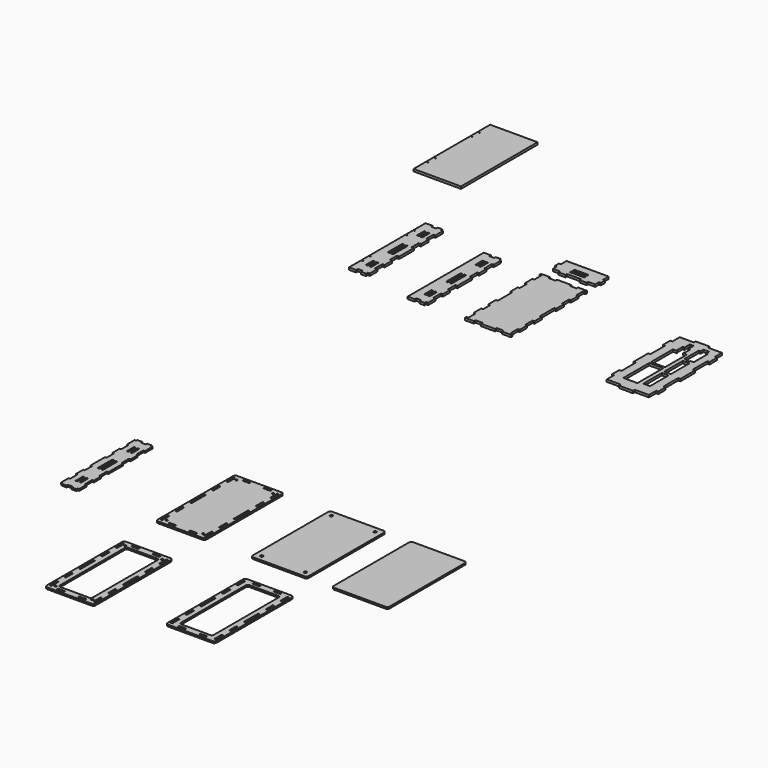
from build123d import *

# Parameters (mm, degrees)
F0_R     = 1.5
F1_DEPTH = 6.33
F0_W     = 40
F0_H     = 5.2
F0_H_2   = 92
F0_W_2   = 19
F0_H_3   = 66
F0_W_3   = 5.2
F0_H_4   = 26
F0_H_5   = 52
F0_R_2   = 2.8
F0_W_4   = 4.5
F0_H_6   = 25.7
F0_H_7   = 25.4
F2_DEPTH = 5
F0_R_3   = 3.8


# Not quite as in the source:
# - ends of sketch curves that miss each other by under 0.0002 mm in the source are joined


with BuildPart() as f1:
    # F0 (on Top) → F1 (new body)
    with BuildSketch(Plane.XY):
        Polygon((-447.6903581619, 704.729092989), (-582.6903581619, 704.729092989), (-582.6903581619, 660.318092989), (-582.6903581619, 432.069092989), (-447.6903581619, 432.069092989), (-447.6903581619, 568.399092989), align=None)
        with Locations((-577.6903581619, 476.480092989)):
            Circle(F0_R, mode=Mode.SUBTRACT)
        with Locations((-577.4039030075, 503.1310149765)):
            Circle(F0_R, mode=Mode.SUBTRACT)
        with BuildLine():
            ThreePointArc((-577.6903581619, 635.218092989), (-576.6296979901, 634.7787531607), (-576.1903581619, 633.718092989))
            ThreePointArc((-576.1903581619, 633.718092989), (-578.7510183337, 632.6574328172), (-577.6903581619, 635.218092989))
        make_face(mode=Mode.SUBTRACT)
        with BuildLine():
            ThreePointArc((-577.6903581619, 658.818092989), (-578.7510183337, 659.2574328172), (-579.1903581619, 660.318092989))
            ThreePointArc((-579.1903581619, 660.318092989), (-577.6903581619, 661.818092989), (-576.1903581619, 660.318092989))
            ThreePointArc((-576.1903581619, 660.318092989), (-576.6296979901, 659.2574328172), (-577.6903581619, 658.818092989))
        make_face(mode=Mode.SUBTRACT)
    extrude(amount=F1_DEPTH)


with BuildPart() as f1b:
    # F0 (on Top) → F1, piece 2 (new body)
    with BuildSketch(Plane.XY):
        Polygon((-0.3, 209.1742812097), (-19.7, 209.1742812097), (-19.7, 214.6742812097), (-45.5, 214.6742812097), (-45.5, 209.1742812097), (-40, 209.1742812097), (-40, 183.4742812097), (-45.5, 183.4742812097), (-45.5, 156.8742812097), (-40, 156.8742812097), (-40, 131.4742812097), (-45.5, 131.4742812097), (-45.5, 104.8742812097), (-40, 104.8742812097), (-40, 79.1742812097), (-40, 53.4742812097), (-45.5, 53.4742812097), (-45.5, 26.8742812097), (-40, 26.8742812097), (-40, 1.4742812097), (-45.5, 1.4742812097), (-45.5, -25.1257187903), (-40, -25.1257187903), (-40, -50.8257187903), (-45.5, -50.8257187903), (-45.5, -56.3257187903), (-19.7, -56.3257187903), (-19.7, -50.8257187903), (-0.3, -50.8257187903), (-0.3, -56.3257187903), (20, -56.3257187903), (40.3, -56.3257187903), (40.3, -50.8257187903), (59.7, -50.8257187903), (59.7, -56.3257187903), (85.5, -56.3257187903), (85.5, -50.8257187903), (80, -50.8257187903), (80, -25.1257187903), (85.5, -25.1257187903), (85.5, 1.4742812097), (80, 1.4742812097), (80, 26.8742812097), (85.5, 26.8742812097), (85.5, 53.4742812097), (80, 53.4742812097), (80, 79.1742812097), (80, 104.8742812097), (85.5, 104.8742812097), (85.5, 131.4742812097), (80, 131.4742812097), (80, 156.8742812097), (85.5, 156.8742812097), (85.5, 183.4742812097), (80, 183.4742812097), (80, 209.1742812097), (85.5, 209.1742812097), (85.5, 214.6742812097), (59.7, 214.6742812097), (59.7, 209.1742812097), (40.3, 209.1742812097), (40.3, 214.6742812097), (20, 214.6742812097), (-0.3, 214.6742812097), align=None)
    extrude(amount=F1_DEPTH)


with BuildPart() as f1c:
    # F0 (on Top) → F1, piece 3 (new body)
    with BuildSketch(Plane.XY):
        Polygon((-40, 263.7736713409), (-40, 250.0736713409), (-20.3, 250.0736713409), (-20, 250.0736713409), (-20, 244.5736713409), (0, 244.5736713409), (0, 250.0736713409), (0.3, 250.0736713409), (20, 250.0736713409), (39.7, 250.0736713409), (40, 250.0736713409), (40, 244.5736713409), (44.012218684, 244.5736713409), (60, 244.5736713409), (60, 250.0736713409), (60.3, 250.0736713409), (80, 250.0736713409), (80, 263.7736713409), (85.5, 263.7736713409), (85.5, 278.3736713409), (80, 278.3736713409), (80, 292.0736713409), (80, 298.4036713409), (60, 298.4036713409), (40, 298.4036713409), (0, 298.4036713409), (-20, 298.4036713409), (-40, 298.4036713409), (-40, 292.0736713409), (-40, 278.3736713409), (-45.5, 278.3736713409), (-45.5, 263.7736713409), align=None)
        with Locations((20, 263.6386713409)):
            Rectangle(F0_W, F0_H, mode=Mode.SUBTRACT)
        with Locations((20, 273.8386713409)):
            Rectangle(F0_W, F0_H, mode=Mode.SUBTRACT)
    extrude(amount=F1_DEPTH)


with BuildPart() as f1d:
    # F0 (on Top) → F1, piece 4 (new body)
    with BuildSketch(Plane.XY):
        Polygon((385.8841769994, -91.011034461), (405.8841769994, -91.011034461), (425.8841769994, -91.011034461), (425.8841769994, -97.341034461), (465.8841769994, -97.341034461), (465.8841769994, -91.011034461), (485.8841769994, -91.011034461), (505.8841769994, -91.011034461), (505.8841769994, -65.011034461), (512.2141769994, -65.011034461), (512.2141769994, -39.011034461), (505.8841769994, -39.011034461), (505.8841769994, -13.011034461), (505.8841769994, 12.988965539), (512.2141769994, 12.988965539), (512.2141769994, 64.988965539), (505.8841769994, 64.988965539), (505.8841769994, 90.988965539), (505.8841769994, 116.988965539), (512.2141769994, 116.988965539), (512.2141769994, 142.988965539), (505.8841769994, 142.988965539), (505.8841769994, 168.988965539), (485.8841769994, 168.988965539), (465.8841769994, 168.988965539), (465.8841769994, 175.318965539), (445.8841769994, 175.318965539), (425.8841769994, 175.318965539), (425.8841769994, 168.988965539), (405.8841769994, 168.988965539), (385.8841769994, 168.988965539), (385.8841769994, 142.988965539), (379.5541769994, 142.988965539), (379.5541769994, 116.988965539), (385.8841769994, 116.988965539), (385.8841769994, 90.988965539), (385.8841769994, 64.988965539), (379.5541769994, 64.988965539), (379.5541769994, 12.988965539), (385.8841769994, 12.988965539), (385.8841769994, -13.011034461), (385.8841769994, -39.011034461), (379.5541769994, -39.011034461), (379.5541769994, -65.011034461), (385.8841769994, -65.011034461), align=None)
        with Locations((430.4254828245, -16.4253961511)):
            Rectangle(F0_W, F0_H_2, mode=Mode.SUBTRACT)
        with Locations((471.857395351, -23.1853164307)):
            Rectangle(F0_W_2, F0_H_3, mode=Mode.SUBTRACT)
        Polygon((424.9906819054, 136.7675569632), (424.9906819054, 155.7675569632), (435.9906819054, 155.7675569632), (435.9906819054, 154.7675569632), (435.9906819054, 136.7675569632), (440.9906819054, 136.7675569632), (440.9906819054, 118.7675569632), (439.4906819054, 118.7675569632), (439.4906819054, 113.7675569632), (450.4906819054, 113.7675569632), (450.4906819054, 35.7675569632), (410.4906819054, 35.7675569632), (410.4906819054, 113.7675569632), (421.4906819054, 113.7675569632), (421.4906819054, 118.7675569632), (419.9906819054, 118.7675569632), (419.9906819054, 136.7675569632), align=None, mode=Mode.SUBTRACT)
        with Locations((471.857395351, 51.1568081991)):
            Rectangle(F0_W_2, F0_H_3, mode=Mode.SUBTRACT)
        Polygon((459.2148857416, 94.0252485254), (459.2148857416, 145.0252485254), (464.2148857416, 145.0252485254), (464.2148857416, 155.0252485254), (472.2148857416, 155.0252485254), (480.2148857416, 155.0252485254), (480.2148857416, 145.0252485254), (485.2148857416, 145.0252485254), (485.2148857416, 94.0252485254), (475.7148857416, 94.0252485254), (475.7148857416, 89.0252485254), (472.2148857416, 89.0252485254), (468.7148857416, 89.0252485254), (468.7148857416, 94.0252485254), align=None, mode=Mode.SUBTRACT)
    extrude(amount=F1_DEPTH)


with BuildPart() as f1e:
    # F0 (on Top) → F1, piece 5 (new body)
    with BuildSketch(Plane.XY):
        Polygon((-181.5613321495, 209.1742812097), (-188.5613321495, 209.1742812097), (-188.5613321495, 214.6742812097), (-208.8913321495, 214.6742812097), (-208.8913321495, 209.1742812097), (-208.8913321495, 183.1742812097), (-208.8913321495, 157.1742812097), (-208.8913321495, 79.1742812097), (-208.8913321495, 1.1742812097), (-208.8913321495, -24.8257187903), (-208.8913321495, -50.8257187903), (-208.8913321495, -56.3257187903), (-188.5613321495, -56.3257187903), (-188.5613321495, -50.8257187903), (-181.5613321495, -50.8257187903), (-174.8613321495, -50.8257187903), (-174.5613321495, -50.8257187903), (-174.5613321495, -56.3257187903), (-160.5613321495, -56.3257187903), (-160.5613321495, -50.8257187903), (-155.0613321495, -50.8257187903), (-155.0613321495, -24.8257187903), (-160.5613321495, -24.8257187903), (-160.5613321495, -24.5257187903), (-160.5613321495, 0.8742812097), (-160.5613321495, 1.1742812097), (-155.0613321495, 1.1742812097), (-155.0613321495, 27.1742812097), (-160.5613321495, 27.1742812097), (-160.5613321495, 27.4742812097), (-160.5613321495, 52.8742812097), (-160.5613321495, 53.1742812097), (-155.0613321495, 53.1742812097), (-155.0613321495, 79.1742812097), (-155.0613321495, 105.1742812097), (-160.5613321495, 105.1742812097), (-160.5613321495, 105.4742812097), (-160.5613321495, 130.8742812097), (-160.5613321495, 131.1742812097), (-155.0613321495, 131.1742812097), (-155.0613321495, 157.1742812097), (-160.5613321495, 157.1742812097), (-160.5613321495, 157.4742812097), (-160.5613321495, 182.8742812097), (-160.5613321495, 183.1742812097), (-155.0613321495, 183.1742812097), (-155.0613321495, 209.4742812097), (-160.2613321495, 209.4742812097), (-160.5613321495, 209.4742812097), (-160.5613321495, 214.6742812097), (-174.5613321495, 214.6742812097), (-174.5613321495, 209.1742812097), (-174.8613321495, 209.1742812097), align=None)
        Polygon((-184.7263321495, -24.8257187903), (-186.9263321495, -24.8257187903), (-186.9263321495, 1.1742812097), (-181.7263321495, 1.1742812097), (-181.7263321495, -24.8257187903), align=None, mode=Mode.SUBTRACT)
        with Locations((-174.1263321495, -11.8257187903)):
            Rectangle(F0_W_3, F0_H_4, mode=Mode.SUBTRACT)
        Polygon((-186.9263321495, 79.1742812097), (-186.9263321495, 105.1742812097), (-181.8263321495, 105.1742812097), (-181.8263321495, 79.1742812097), (-181.8263321495, 53.1742812097), (-186.9263321495, 53.1742812097), align=None, mode=Mode.SUBTRACT)
        Polygon((-176.7263321495, 105.1742812097), (-171.6263321495, 105.1742812097), (-171.6263321495, 79.1742812097), (-171.6263321495, 53.1742812097), (-176.7263321495, 53.1742812097), (-176.7263321495, 79.1742812097), align=None, mode=Mode.SUBTRACT)
        Polygon((-186.9263321495, 157.1742812097), (-186.9263321495, 183.1742812097), (-184.7263321495, 183.1742812097), (-181.7263321495, 183.1742812097), (-181.7263321495, 157.1742812097), align=None, mode=Mode.SUBTRACT)
        with Locations((-174.1263321495, 170.1742812097)):
            Rectangle(F0_W_3, F0_H_4, mode=Mode.SUBTRACT)
    extrude(amount=F1_DEPTH)


with BuildPart() as f1f:
    # F0 (on Top) → F1, piece 6 (new body)
    with BuildSketch(Plane.XY):
        Polygon((-371.3439686881, 239.1072111412), (-378.3439686881, 239.1072111412), (-378.3439686881, 244.8072111412), (-398.6739686881, 244.8072111412), (-398.6739686881, 239.1072111412), (-398.6739686881, 212.5072111412), (-398.6739686881, 200.4259941339), (-398.6739686881, 186.5072111412), (-398.6739686881, 173.8259941339), (-398.6739686881, -21.4927888588), (-398.6739686881, -27.8227888588), (-392.3439686881, -27.8227888588), (-378.3439686881, -27.8227888588), (-378.3439686881, -21.4927888588), (-364.6439686881, -21.4927888588), (-364.6439686881, -27.8227888588), (-364.3439686881, -27.8227888588), (-357.3439686881, -27.8227888588), (-350.3439686881, -27.8227888588), (-350.0439686881, -27.8227888588), (-350.0439686881, -21.4927888588), (-344.0139686881, -21.4927888588), (-344.0139686881, 4.5072111412), (-350.3439686881, 4.5072111412), (-350.3439686881, 4.8072111412), (-350.3439686881, 30.2072111412), (-350.3439686881, 30.5072111412), (-344.0139686881, 30.5072111412), (-344.0139686881, 56.5072111412), (-350.3439686881, 56.5072111412), (-350.3439686881, 56.8072111412), (-350.3439686881, 82.2072111412), (-350.3439686881, 82.5072111412), (-344.0139686881, 82.5072111412), (-344.0139686881, 108.5072111412), (-344.0139686881, 134.5072111412), (-350.3439686881, 134.5072111412), (-350.3439686881, 134.8072111412), (-350.3439686881, 159.6072111412), (-350.3439686881, 159.9072111412), (-344.0139686881, 159.9072111412), (-344.0139686881, 186.5072111412), (-350.3439686881, 186.5072111412), (-350.3439686881, 186.8072111412), (-350.3439686881, 212.5072111412), (-344.8439686881, 212.5072111412), (-344.8439686881, 239.1072111412), (-350.0439686881, 239.1072111412), (-350.3439686881, 239.1072111412), (-350.3439686881, 244.8072111412), (-364.3439686881, 244.8072111412), (-364.3439686881, 239.1072111412), (-364.6439686881, 239.1072111412), align=None)
        with Locations((-394.6739686881, 16.5884281485)):
            Circle(F0_R, mode=Mode.SUBTRACT)
        with Locations((-374.1089686881, 17.5072111412)):
            Rectangle(F0_W_3, F0_H_4, mode=Mode.SUBTRACT)
        with Locations((-394.6739686881, 43.1884281485)):
            Circle(F0_R, mode=Mode.SUBTRACT)
        with Locations((-363.9089686881, 17.5072111412)):
            Rectangle(F0_W_3, F0_H_4, mode=Mode.SUBTRACT)
        with Locations((-374.1089686881, 108.5072111412)):
            Rectangle(F0_W_3, F0_H_5, mode=Mode.SUBTRACT)
        with Locations((-363.9089686881, 108.5072111412)):
            Rectangle(F0_W_3, F0_H_5, mode=Mode.SUBTRACT)
        with BuildLine():
            ThreePointArc((-393.1739686881, 173.8259941339), (-394.6739686881, 172.3259941339), (-396.1739686881, 173.8259941339))
            ThreePointArc((-396.1739686881, 173.8259941339), (-395.7346288598, 174.8866543057), (-394.6739686881, 175.3259941339))
            ThreePointArc((-394.6739686881, 175.3259941339), (-393.6133085163, 174.8866543057), (-393.1739686881, 173.8259941339))
        make_face(mode=Mode.SUBTRACT)
        with BuildLine():
            ThreePointArc((-394.6739686881, 198.9259941339), (-395.7346288598, 199.3653339622), (-396.1739686881, 200.4259941339))
            ThreePointArc((-396.1739686881, 200.4259941339), (-394.6739686881, 201.9259941339), (-393.1739686881, 200.4259941339))
            ThreePointArc((-393.1739686881, 200.4259941339), (-393.6133085163, 199.3653339622), (-394.6739686881, 198.9259941339))
        make_face(mode=Mode.SUBTRACT)
        Polygon((-376.7089686881, 186.5072111412), (-376.7089686881, 212.5072111412), (-374.5089686881, 212.5072111412), (-371.5089686881, 212.5072111412), (-371.5089686881, 186.5072111412), align=None, mode=Mode.SUBTRACT)
        with Locations((-363.9089686881, 199.5072111412)):
            Rectangle(F0_W_3, F0_H_4, mode=Mode.SUBTRACT)
    extrude(amount=F1_DEPTH)


with BuildPart() as f2:
    # F0 (on Top) → F2 (new body)
    with BuildSketch(Plane.XY):
        with BuildLine():
            Line((26.3501927257, -971.6120737515), (26.3501927257, -1105.7620737515))
            Line((26.3501927257, -1105.7620737515), (26.3501927257, -1239.9120737515))
            ThreePointArc((26.3501927257, -1239.9120737515), (28.2100646651, -1244.402201812), (32.7001927257, -1246.2620737515))
            Line((32.7001927257, -1246.2620737515), (95.8501927257, -1246.2620737515))
            Line((95.8501927257, -1246.2620737515), (159.0001927257, -1246.2620737515))
            ThreePointArc((159.0001927257, -1246.2620737515), (163.4903207862, -1244.402201812), (165.3501927257, -1239.9120737515))
            Line((165.3501927257, -1239.9120737515), (165.3501927257, -1105.7620737515))
            Line((165.3501927257, -1105.7620737515), (165.3501927257, -971.6120737515))
            ThreePointArc((165.3501927257, -971.6120737515), (163.4903207862, -967.121945691), (159.0001927257, -965.2620737515))
            Line((159.0001927257, -965.2620737515), (95.8501927257, -965.2620737515))
            Line((95.8501927257, -965.2620737515), (32.7001927257, -965.2620737515))
            ThreePointArc((32.7001927257, -965.2620737515), (28.2100646651, -967.121945691), (26.3501927257, -971.6120737515))
        make_face()
        with Locations((43.6520688236, -1229.9456782266)):
            Circle(F0_R_2, mode=Mode.SUBTRACT)
        with Locations((33.6001927257, -1222.9120737515)):
            Rectangle(F0_W_4, F0_H_6, mode=Mode.SUBTRACT)
        Polygon((75.8501927257, -1236.7620737515), (75.8501927257, -1240.2620737515), (66.2648080312, -1240.2620737515), (55.8501929045, -1240.2620737515), (55.8501927257, -1236.7620737515), (55.8501929045, -1235.7620737515), (65.9648080312, -1235.7620737515), (66.2648080312, -1235.7620737515), (75.8501929045, -1235.7620737515), align=None, mode=Mode.SUBTRACT)
        with Locations((33.6001927257, -1170.7620737515)):
            Rectangle(F0_W_4, F0_H_7, mode=Mode.SUBTRACT)
        Polygon((35.8501927257, -1080.0620737515), (35.8501927257, -1105.7620737515), (35.8501927257, -1131.4620737515), (31.3501927257, -1131.4620737515), (31.3501927257, -1105.7620737515), (31.3501927257, -1080.0620737515), align=None, mode=Mode.SUBTRACT)
        Polygon((125.435577599, -1240.2620737515), (115.8501927257, -1240.2620737515), (115.8501927257, -1236.7620737515), (115.8501927257, -1235.7620737515), (125.435577599, -1235.7620737515), (125.735577599, -1235.7620737515), (135.8501927257, -1235.7620737515), (135.8501927257, -1236.7620737515), (135.8501927257, -1240.2620737515), align=None, mode=Mode.SUBTRACT)
        with Locations((148.0483166277, -1229.9456782266)):
            Circle(F0_R_2, mode=Mode.SUBTRACT)
        with Locations((158.1001927257, -1222.9120737515)):
            Rectangle(F0_W_4, F0_H_6, mode=Mode.SUBTRACT)
        with Locations((158.1001927257, -1170.7620737515)):
            Rectangle(F0_W_4, F0_H_7, mode=Mode.SUBTRACT)
        Polygon((160.3501927257, -1080.0620737515), (160.3501927257, -1105.7620737515), (160.3501927257, -1131.4620737515), (155.8501927257, -1131.4620737515), (155.8501927257, -1105.7620737515), (155.8501927257, -1080.0620737515), align=None, mode=Mode.SUBTRACT)
        with Locations((33.6001927257, -1040.7620737515)):
            Rectangle(F0_W_4, F0_H_7, mode=Mode.SUBTRACT)
        with Locations((33.6001927257, -988.6120737515)):
            Rectangle(F0_W_4, F0_H_6, mode=Mode.SUBTRACT)
        with Locations((43.6520688236, -981.5784692764)):
            Circle(F0_R_2, mode=Mode.SUBTRACT)
        Polygon((75.8501929045, -975.7620737515), (66.2648080312, -975.7620737515), (65.9648080312, -975.7620737515), (55.8501929045, -975.7620737515), (55.8501929045, -971.2620737515), (66.2648080312, -971.2620737515), (75.8501929045, -971.2620737515), align=None, mode=Mode.SUBTRACT)
        with Locations((158.1001927257, -1040.7620737515)):
            Rectangle(F0_W_4, F0_H_7, mode=Mode.SUBTRACT)
        with Locations((158.1001927257, -988.6120737515)):
            Rectangle(F0_W_4, F0_H_6, mode=Mode.SUBTRACT)
        Polygon((115.8501927257, -975.7620737515), (115.8501927257, -971.2620737515), (125.435577599, -971.2620737515), (135.8501927257, -971.2620737515), (135.8501927257, -975.7620737515), (125.735577599, -975.7620737515), (125.435577599, -975.7620737515), align=None, mode=Mode.SUBTRACT)
        with Locations((148.0483166277, -981.5784692764)):
            Circle(F0_R_2, mode=Mode.SUBTRACT)
    extrude(amount=F2_DEPTH)


with BuildPart() as f2b:
    # F0 (on Top) → F2, piece 2 (new body)
    with BuildSketch(Plane.XY):
        Polygon((-227.4993014006, -973.8982943573), (-234.4993014006, -973.8982943573), (-234.4993014006, -969.3982943573), (-248.4993014003, -969.3982943573), (-248.4993014003, -973.5982943573), (-248.7993014005, -973.5982943573), (-250.3293014003, -973.5982943573), (-252.9993014008, -973.5982943573), (-252.9993014008, -999.8982943573), (-250.3293014003, -999.8982943573), (-248.4993014007, -999.8982943573), (-248.4993014007, -1000.1982943573), (-248.4993014007, -1025.5982943586), (-248.4993014007, -1025.8982943573), (-252.9993014008, -1025.8982943573), (-252.9993014008, -1051.8982943587), (-248.4993014007, -1051.8982943587), (-248.4993014007, -1052.1982943586), (-248.4993014007, -1077.5982943586), (-248.4993014007, -1077.8982943578), (-252.9993014008, -1077.8982943578), (-252.9993014008, -1103.8982943586), (-252.9993014008, -1129.8982943594), (-248.4993014007, -1129.8982943594), (-248.4993014007, -1130.1982943586), (-248.4993014007, -1155.5982943586), (-248.4993014007, -1155.8982943586), (-252.9993014008, -1155.8982943586), (-252.9993014008, -1181.8982943599), (-248.4993014007, -1181.8982943599), (-248.4993014007, -1182.1982943587), (-248.4993014007, -1207.5982943573), (-248.4993014007, -1207.8982943599), (-252.9993014008, -1207.8982943599), (-252.9993014008, -1234.1982943599), (-248.7993014005, -1234.1982943599), (-248.4993014003, -1234.1982943599), (-248.4993014003, -1238.3982943599), (-234.4993014006, -1238.3982943599), (-234.4993014006, -1233.8982943599), (-227.4993014006, -1233.8982943599), (-220.7993014006, -1233.8982943599), (-220.4993014006, -1233.8982943599), (-220.1993014006, -1233.8982943599), (-220.1993014006, -1238.3982943599), (-206.4993014008, -1238.3982943599), (-206.4993014008, -1234.1982943599), (-206.1993014006, -1234.1982943599), (-201.9993014004, -1234.1982943599), (-201.9993014004, -1207.8982943599), (-206.4993014004, -1207.8982943599), (-206.4993014004, -1207.5982943599), (-206.4993014004, -1182.1982943586), (-206.4993014004, -1181.8982943599), (-201.9993014004, -1181.8982943599), (-201.9993014004, -1155.8982943586), (-206.4993014004, -1155.8982943586), (-206.4993014004, -1155.5982943586), (-206.4993014004, -1130.1982943586), (-206.4993014004, -1129.8982943594), (-201.9993014004, -1129.8982943594), (-201.9993014004, -1103.8982943586), (-201.9993014004, -1077.8982943578), (-206.4993014004, -1077.8982943578), (-206.4993014004, -1077.5982943586), (-206.4993014004, -1052.1982943586), (-206.4993014004, -1051.8982943587), (-201.9993014004, -1051.8982943587), (-201.9993014004, -1025.8982943573), (-206.4993014004, -1025.8982943573), (-206.4993014004, -1025.5982943585), (-206.4993014004, -1000.1982943599), (-206.4993014004, -999.8982943573), (-201.9993014004, -999.8982943573), (-201.9993014004, -973.5982943573), (-206.1993014006, -973.5982943573), (-206.4993014008, -973.5982943573), (-206.4993014008, -969.3982943573), (-220.1993014006, -969.3982943573), (-220.1993014006, -973.8982943573), (-220.4993014006, -973.8982943573), (-220.7993014006, -973.8982943573), align=None)
        Polygon((-228.3643014004, -1181.8982943599), (-228.3643014004, -1207.8982943599), (-229.1643014004, -1207.8982943599), (-230.6643014004, -1207.8982943599), (-232.8643014004, -1207.8982943599), (-232.8643014004, -1181.8982943599), align=None, mode=Mode.SUBTRACT)
        Polygon((-228.3643014004, -1077.8982943573), (-228.3643014004, -1103.8982943586), (-228.3643014004, -1129.8982943599), (-232.8643014004, -1129.8982943599), (-232.8643014004, -1103.8982943586), (-232.8643014004, -1077.8982943573), align=None, mode=Mode.SUBTRACT)
        with Locations((-220.4143014004, -1194.8982943599)):
            Rectangle(F0_W_4, F0_H_4, mode=Mode.SUBTRACT)
        Polygon((-218.1643014004, -1077.8982943573), (-218.1643014004, -1103.8982943586), (-218.1643014004, -1129.8982943599), (-222.6643014004, -1129.8982943599), (-222.6643014004, -1103.8982943586), (-222.6643014004, -1077.8982943573), align=None, mode=Mode.SUBTRACT)
        Polygon((-232.8643014004, -1025.8982943573), (-232.8643014004, -999.8982943573), (-230.6643014004, -999.8982943573), (-229.1643014004, -999.8982943573), (-228.3643014004, -999.8982943573), (-228.3643014004, -1025.8982943573), align=None, mode=Mode.SUBTRACT)
        with Locations((-220.4143014004, -1012.8982943573)):
            Rectangle(F0_W_4, F0_H_4, mode=Mode.SUBTRACT)
    extrude(amount=F2_DEPTH)


with BuildPart() as f2c:
    # F0 (on Top) → F2, piece 3 (new body)
    with BuildSketch(Plane.XY):
        with BuildLine():
            Line((378.8151222394, -967.972550389), (305.5505071127, -967.972550389))
            ThreePointArc((305.5505071127, -967.972550389), (301.0603790522, -969.8324223285), (299.2005071127, -974.322550389))
            Line((299.2005071127, -974.322550389), (299.2005071127, -1108.472550389))
            Line((299.2005071127, -1108.472550389), (299.2005071127, -1242.622550389))
            ThreePointArc((299.2005071127, -1242.622550389), (301.0603790522, -1247.1126784496), (305.5505071127, -1248.972550389))
            Line((305.5505071127, -1248.972550389), (378.8151222394, -1248.972550389))
            Line((378.8151222394, -1248.972550389), (452.0797373661, -1248.972550389))
            ThreePointArc((452.0797373661, -1248.972550389), (456.5698654266, -1247.1126784496), (458.4297373661, -1242.622550389))
            Line((458.4297373661, -1242.622550389), (458.4297373661, -1108.472550389))
            Line((458.4297373661, -1108.472550389), (458.4297373661, -974.322550389))
            ThreePointArc((458.4297373661, -974.322550389), (456.5698654266, -969.8324223285), (452.0797373661, -967.972550389))
            Line((452.0797373661, -967.972550389), (378.8151222394, -967.972550389))
        make_face()
        with Locations((316.5023832107, -1232.6561548641)):
            Circle(F0_R_3, mode=Mode.SUBTRACT)
        with Locations((441.1278612682, -1232.6561548641)):
            Circle(F0_R_3, mode=Mode.SUBTRACT)
        with Locations((316.5023832107, -984.288945914)):
            Circle(F0_R_3, mode=Mode.SUBTRACT)
        with Locations((441.1278612682, -984.288945914)):
            Circle(F0_R_3, mode=Mode.SUBTRACT)
    extrude(amount=F2_DEPTH)


with BuildPart() as f2d:
    # F0 (on Top) → F2, piece 4 (new body)
    with BuildSketch(Plane.XY):
        with BuildLine():
            Line((611.0029862519, -970.2220103933), (537.7383711252, -970.2220103933))
            ThreePointArc((537.7383711252, -970.2220103933), (533.2482430646, -972.0818823327), (531.3883711252, -976.5720103933))
            Line((531.3883711252, -976.5720103933), (531.3883711252, -1110.7220103933))
            Line((531.3883711252, -1110.7220103933), (531.3883711252, -1244.8720103933))
            ThreePointArc((531.3883711252, -1244.8720103933), (533.2482430646, -1249.3621384538), (537.7383711252, -1251.2220103933))
            Line((537.7383711252, -1251.2220103933), (611.0029862519, -1251.2220103933))
            Line((611.0029862519, -1251.2220103933), (684.2676013785, -1251.2220103933))
            ThreePointArc((684.2676013785, -1251.2220103933), (688.7577294391, -1249.3621384538), (690.6176013785, -1244.8720103933))
            Line((690.6176013785, -1244.8720103933), (690.6176013785, -1110.7220103933))
            Line((690.6176013785, -1110.7220103933), (690.6176013785, -976.5720103933))
            ThreePointArc((690.6176013785, -976.5720103933), (688.7577294391, -972.0818823327), (684.2676013785, -970.2220103933))
            Line((684.2676013785, -970.2220103933), (611.0029862519, -970.2220103933))
        make_face()
    extrude(amount=F2_DEPTH)


with BuildPart() as f2e:
    # F0 (on Top) → F2, piece 5 (new body)
    with BuildSketch(Plane.XY):
        with BuildLine():
            Line((354.3367418902, -1345.9159692793), (354.3367418902, -1480.0659692793))
            Line((354.3367418902, -1480.0659692793), (354.3367418902, -1614.2159692793))
            ThreePointArc((354.3367418902, -1614.2159692793), (356.1966138296, -1618.7060973398), (360.6867418902, -1620.5659692793))
            Line((360.6867418902, -1620.5659692793), (423.8367418902, -1620.5659692793))
            Line((423.8367418902, -1620.5659692793), (486.9867418902, -1620.5659692793))
            ThreePointArc((486.9867418902, -1620.5659692793), (491.4768699507, -1618.7060973398), (493.3367418902, -1614.2159692793))
            Line((493.3367418902, -1614.2159692793), (493.3367418902, -1480.0659692793))
            Line((493.3367418902, -1480.0659692793), (493.3367418902, -1345.9159692793))
            ThreePointArc((493.3367418902, -1345.9159692793), (491.4768699507, -1341.4258412187), (486.9867418902, -1339.5659692793))
            Line((486.9867418902, -1339.5659692793), (423.8367418902, -1339.5659692793))
            Line((423.8367418902, -1339.5659692793), (360.6867418902, -1339.5659692793))
            ThreePointArc((360.6867418902, -1339.5659692793), (356.1966138296, -1341.4258412187), (354.3367418902, -1345.9159692793))
        make_face()
        with Locations((361.5867418902, -1597.2159692793)):
            Rectangle(F0_W_4, F0_H_6, mode=Mode.SUBTRACT)
        with Locations((361.5867418902, -1545.0659692793)):
            Rectangle(F0_W_4, F0_H_7, mode=Mode.SUBTRACT)
        Polygon((403.8367418902, -1611.0659692793), (403.8367418902, -1614.5659692793), (394.2513571957, -1614.5659692793), (383.836742069, -1614.5659692793), (383.8367418902, -1611.0659692793), (383.836742069, -1610.0659692793), (393.9513571957, -1610.0659692793), (394.2513571957, -1610.0659692793), (403.836742069, -1610.0659692793), align=None, mode=Mode.SUBTRACT)
        Polygon((453.4221267635, -1614.5659692793), (443.8367418902, -1614.5659692793), (443.8367418902, -1611.0659692793), (443.8367418902, -1610.0659692793), (453.4221267635, -1610.0659692793), (453.7221267635, -1610.0659692793), (463.8367418902, -1610.0659692793), (463.8367418902, -1611.0659692793), (463.8367418902, -1614.5659692793), align=None, mode=Mode.SUBTRACT)
        with Locations((486.0867418902, -1597.2159692793)):
            Rectangle(F0_W_4, F0_H_6, mode=Mode.SUBTRACT)
        with Locations((486.0867418902, -1545.0659692793)):
            Rectangle(F0_W_4, F0_H_7, mode=Mode.SUBTRACT)
        Polygon((363.8367418902, -1454.3659692793), (363.8367418902, -1480.0659692793), (363.8367418902, -1505.7659692793), (359.3367418902, -1505.7659692793), (359.3367418902, -1480.0659692793), (359.3367418902, -1454.3659692793), align=None, mode=Mode.SUBTRACT)
        with Locations((361.5867418902, -1415.0659692793)):
            Rectangle(F0_W_4, F0_H_7, mode=Mode.SUBTRACT)
        with Locations((361.5867418902, -1362.9159692793)):
            Rectangle(F0_W_4, F0_H_6, mode=Mode.SUBTRACT)
        with BuildLine():
            Line((465.6188140279, -1601.0418546776), (423.8367418902, -1601.0418546776))
            Line((423.8367418902, -1601.0418546776), (382.0546697524, -1601.0418546776))
            ThreePointArc((382.0546697524, -1601.0418546776), (378.5191358465, -1599.5773885835), (377.0546697524, -1596.0418546776))
            Line((377.0546697524, -1596.0418546776), (377.0546697524, -1480.0659692793))
            Line((377.0546697524, -1480.0659692793), (377.0546697524, -1364.090083881))
            ThreePointArc((377.0546697524, -1364.090083881), (378.5191358465, -1360.5545499751), (382.0546697524, -1359.090083881))
            Line((382.0546697524, -1359.090083881), (423.8367418902, -1359.090083881))
            Line((423.8367418902, -1359.090083881), (465.6188140279, -1359.090083881))
            ThreePointArc((465.6188140279, -1359.090083881), (469.1543479338, -1360.5545499751), (470.6188140279, -1364.090083881))
            Line((470.6188140279, -1364.090083881), (470.6188140279, -1480.0659692793))
            Line((470.6188140279, -1480.0659692793), (470.6188140279, -1596.0418546776))
            ThreePointArc((470.6188140279, -1596.0418546776), (469.1543479338, -1599.5773885835), (465.6188140279, -1601.0418546776))
        make_face(mode=Mode.SUBTRACT)
        Polygon((488.3367418902, -1454.3659692793), (488.3367418902, -1480.0659692793), (488.3367418902, -1505.7659692793), (483.8367418902, -1505.7659692793), (483.8367418902, -1480.0659692793), (483.8367418902, -1454.3659692793), align=None, mode=Mode.SUBTRACT)
        with Locations((486.0867418902, -1415.0659692793)):
            Rectangle(F0_W_4, F0_H_7, mode=Mode.SUBTRACT)
        with Locations((486.0867418902, -1362.9159692793)):
            Rectangle(F0_W_4, F0_H_6, mode=Mode.SUBTRACT)
        Polygon((403.836742069, -1350.0659692793), (394.2513571957, -1350.0659692793), (393.9513571957, -1350.0659692793), (383.836742069, -1350.0659692793), (383.836742069, -1345.5659692793), (394.2513571957, -1345.5659692793), (403.836742069, -1345.5659692793), align=None, mode=Mode.SUBTRACT)
        Polygon((443.8367418902, -1350.0659692793), (443.8367418902, -1345.5659692793), (453.4221267635, -1345.5659692793), (463.8367418902, -1345.5659692793), (463.8367418902, -1350.0659692793), (453.7221267635, -1350.0659692793), (453.4221267635, -1350.0659692793), align=None, mode=Mode.SUBTRACT)
    extrude(amount=F2_DEPTH)


with BuildPart() as f2f:
    # F0 (on Top) → F2, piece 6 (new body)
    with BuildSketch(Plane.XY):
        with BuildLine():
            Line((31.7402544428, -1373.5117336344), (31.7402544428, -1507.6617336344))
            Line((31.7402544428, -1507.6617336344), (31.7402544428, -1641.8117336344))
            ThreePointArc((31.7402544428, -1641.8117336344), (33.6001263823, -1646.3018616949), (38.0902544428, -1648.1617336344))
            Line((38.0902544428, -1648.1617336344), (101.2402544428, -1648.1617336344))
            Line((101.2402544428, -1648.1617336344), (164.3902544428, -1648.1617336344))
            ThreePointArc((164.3902544428, -1648.1617336344), (168.8803825034, -1646.3018616949), (170.7402544428, -1641.8117336344))
            Line((170.7402544428, -1641.8117336344), (170.7402544428, -1507.6617336344))
            Line((170.7402544428, -1507.6617336344), (170.7402544428, -1373.5117336344))
            ThreePointArc((170.7402544428, -1373.5117336344), (168.8803825034, -1369.0216055738), (164.3902544428, -1367.1617336344))
            Line((164.3902544428, -1367.1617336344), (101.2402544428, -1367.1617336344))
            Line((101.2402544428, -1367.1617336344), (38.0902544428, -1367.1617336344))
            ThreePointArc((38.0902544428, -1367.1617336344), (33.6001263823, -1369.0216055738), (31.7402544428, -1373.5117336344))
        make_face()
        with Locations((49.0421305408, -1631.8453381094)):
            Circle(F0_R_2, mode=Mode.SUBTRACT)
        with Locations((38.9902544428, -1624.8117336344)):
            Rectangle(F0_W_4, F0_H_6, mode=Mode.SUBTRACT)
        Polygon((81.2402544428, -1638.6617336344), (81.2402544428, -1642.1617336344), (71.6548697483, -1642.1617336344), (61.2402546216, -1642.1617336344), (61.2402544428, -1638.6617336344), (61.2402546216, -1637.6617336344), (71.3548697483, -1637.6617336344), (71.6548697483, -1637.6617336344), (81.2402546216, -1637.6617336344), align=None, mode=Mode.SUBTRACT)
        with Locations((38.9902544428, -1572.6617336344)):
            Rectangle(F0_W_4, F0_H_7, mode=Mode.SUBTRACT)
        Polygon((41.2402544428, -1481.9617336344), (41.2402544428, -1507.6617336344), (41.2402544428, -1533.3617336344), (36.7402544428, -1533.3617336344), (36.7402544428, -1507.6617336344), (36.7402544428, -1481.9617336344), align=None, mode=Mode.SUBTRACT)
        with Locations((38.9902544428, -1442.6617336344)):
            Rectangle(F0_W_4, F0_H_7, mode=Mode.SUBTRACT)
        with Locations((38.9902544428, -1390.5117336344)):
            Rectangle(F0_W_4, F0_H_6, mode=Mode.SUBTRACT)
        with Locations((49.0421305408, -1383.4781291593)):
            Circle(F0_R_2, mode=Mode.SUBTRACT)
        Polygon((81.2402546216, -1377.6617336344), (71.6548697483, -1377.6617336344), (71.3548697483, -1377.6617336344), (61.2402546216, -1377.6617336344), (61.2402546216, -1373.1617336344), (71.6548697483, -1373.1617336344), (81.2402546216, -1373.1617336344), align=None, mode=Mode.SUBTRACT)
        Polygon((130.8256393161, -1642.1617336344), (121.2402544428, -1642.1617336344), (121.2402544428, -1638.6617336344), (121.2402544428, -1637.6617336344), (130.8256393161, -1637.6617336344), (131.1256393161, -1637.6617336344), (141.2402544428, -1637.6617336344), (141.2402544428, -1638.6617336344), (141.2402544428, -1642.1617336344), align=None, mode=Mode.SUBTRACT)
        with Locations((153.4383783449, -1631.8453381094)):
            Circle(F0_R_2, mode=Mode.SUBTRACT)
        with Locations((163.4902544428, -1624.8117336344)):
            Rectangle(F0_W_4, F0_H_6, mode=Mode.SUBTRACT)
        with BuildLine():
            Line((143.0223265806, -1628.6376190326), (101.2402544428, -1628.6376190326))
            Line((101.2402544428, -1628.6376190326), (59.4581823051, -1628.6376190326))
            ThreePointArc((59.4581823051, -1628.6376190326), (55.9226483992, -1627.1731529386), (54.4581823051, -1623.6376190326))
            Line((54.4581823051, -1623.6376190326), (54.4581823051, -1507.6617336344))
            Line((54.4581823051, -1507.6617336344), (54.4581823051, -1391.6858482361))
            ThreePointArc((54.4581823051, -1391.6858482361), (55.9226483992, -1388.1503143302), (59.4581823051, -1386.6858482361))
            Line((59.4581823051, -1386.6858482361), (101.2402544428, -1386.6858482361))
            Line((101.2402544428, -1386.6858482361), (143.0223265806, -1386.6858482361))
            ThreePointArc((143.0223265806, -1386.6858482361), (146.5578604865, -1388.1503143302), (148.0223265806, -1391.6858482361))
            Line((148.0223265806, -1391.6858482361), (148.0223265806, -1507.6617336344))
            Line((148.0223265806, -1507.6617336344), (148.0223265806, -1623.6376190326))
            ThreePointArc((148.0223265806, -1623.6376190326), (146.5578604865, -1627.1731529386), (143.0223265806, -1628.6376190326))
        make_face(mode=Mode.SUBTRACT)
        with Locations((163.4902544428, -1572.6617336344)):
            Rectangle(F0_W_4, F0_H_7, mode=Mode.SUBTRACT)
        Polygon((165.7402544428, -1481.9617336344), (165.7402544428, -1507.6617336344), (165.7402544428, -1533.3617336344), (161.2402544428, -1533.3617336344), (161.2402544428, -1507.6617336344), (161.2402544428, -1481.9617336344), align=None, mode=Mode.SUBTRACT)
        with Locations((163.4902544428, -1442.6617336344)):
            Rectangle(F0_W_4, F0_H_7, mode=Mode.SUBTRACT)
        Polygon((121.2402544428, -1377.6617336344), (121.2402544428, -1373.1617336344), (130.8256393161, -1373.1617336344), (141.2402544428, -1373.1617336344), (141.2402544428, -1377.6617336344), (131.1256393161, -1377.6617336344), (130.8256393161, -1377.6617336344), align=None, mode=Mode.SUBTRACT)
        with Locations((153.4383783449, -1383.4781291593)):
            Circle(F0_R_2, mode=Mode.SUBTRACT)
        with Locations((163.4902544428, -1390.5117336344)):
            Rectangle(F0_W_4, F0_H_6, mode=Mode.SUBTRACT)
    extrude(amount=F2_DEPTH)


solid = Compound([f1.part, f1b.part, f1c.part, f1d.part, f1e.part, f1f.part, f2.part, f2b.part, f2c.part, f2d.part, f2e.part, f2f.part])
